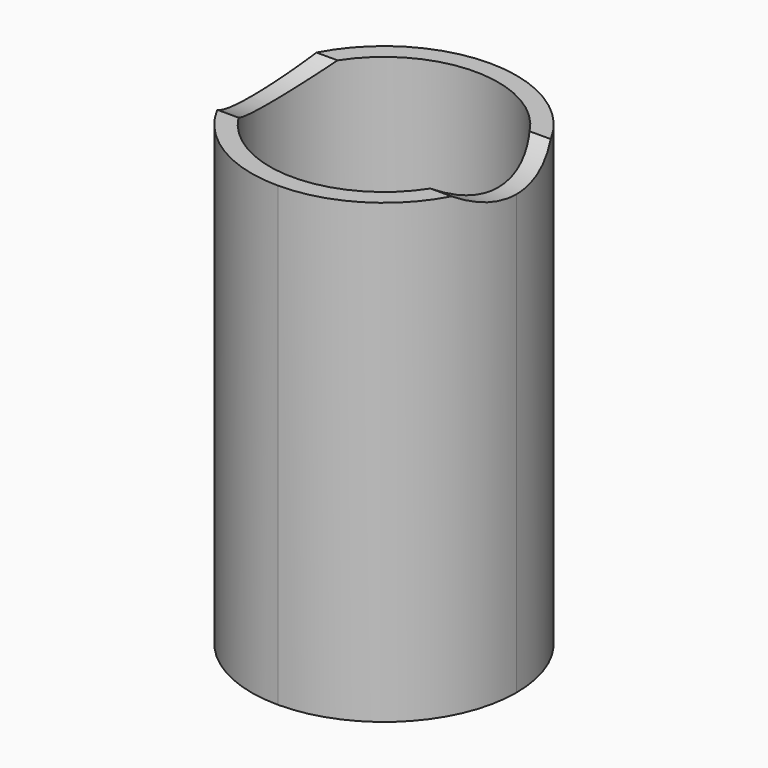
from build123d import *

# Parameters (mm, degrees)
F0_W     = 3.683
F0_H     = 3.683
F0_R     = 1.5875
F1_DEPTH = 6.35
F3_DEPTH = 3.683
F4_R     = 1.84149


# Not quite as in the source:
# - a fillet or chamfer is up to 0.001 mm smaller than in the source, because OpenCascade refuses the exact size


with BuildPart() as f1:
    # F0 (on Top) → F1 (new body)
    with BuildSketch(Plane.XY):
        Rectangle(F0_W, F0_H)
        Circle(F0_R, mode=Mode.SUBTRACT)
    extrude(amount=F1_DEPTH)

    # F2 (on face) → F3 (cut, through all)
    with BuildSketch(Plane.YZ.offset(1.8415)):
        with BuildLine():
            Line((0.8613559079, 6.35), (-0.8613559079, 6.35))
            ThreePointArc((-0.8613559079, 6.35), (0, 6.096), (0.8613559079, 6.35))
        make_face()
    extrude(amount=-F3_DEPTH, mode=Mode.SUBTRACT)

    # F4 (radius 1.8415 in the source; OpenCascade refuses exactly that, so slightly less here)
    f4_edges = [f1.edges().sort_by_distance(p)[0] for p in [
        (-1.8415, -1.8415, 3.175),
        (1.8415, -1.8415, 3.175),
        (-1.8415, 1.8415, 3.175),
        (1.8415, 1.8415, 3.175),
    ]]
    fillet(f4_edges, radius=F4_R)


solid = f1.part
